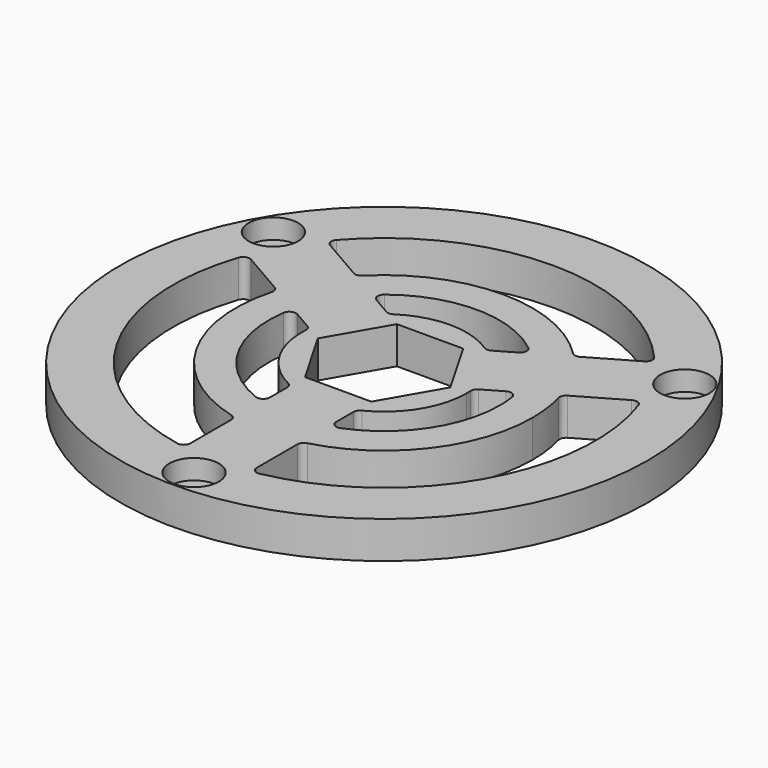
from build123d import *

# Parameters (mm, degrees)
F0_R     = 50.8
F1_DEPTH = 7.14375
F3_DEPTH = 7.14475
F4_R     = 1.27
F5_R     = 4.7625
F6_DEPTH = 3.81


with BuildPart() as f1:
    # F0 (on Top) → F1 (new body)
    with BuildSketch(Plane.XY):
        Circle(F0_R)
        Polygon((-12.7582862486, 0), (-6.3791431243, 11.049), (6.3791431243, 11.049), (12.7582862486, 0), (6.3791431243, -11.049), (-6.3791431243, -11.049), align=None, mode=Mode.SUBTRACT)
    extrude(amount=F1_DEPTH)

    # F2 (on face) → F3 (cut, through all)
    with BuildSketch(Plane.XY.offset(7.14375)):
        with BuildLine():
            Line((-6.3791431243, -40.1362197149), (-6.3791431243, -27.8538535575))
            ThreePointArc((-6.3791431243, -27.8538535575), (-24.7466759131, -14.2875), (-27.3117163362, 8.4024267787))
            Line((-27.3117163362, 8.4024267787), (-37.9485574471, 14.5436098574))
            ThreePointArc((-37.9485574471, 14.5436098574), (-35.1952724098, -20.32), (-6.3791431243, -40.1362197149))
        make_face()
        Polygon((-38.3481822298, 25.019), (-40.8411806922, 25.019), (-42.0876799234, 22.86), (-40.8411806922, 20.701), (-38.3481822298, 20.701), (-37.1016829987, 22.86), align=None)
        Polygon((1.2464992312, -43.561), (-1.2464992312, -43.561), (-2.4929984624, -45.72), (-1.2464992312, -47.879), (1.2464992312, -47.879), (2.4929984624, -45.72), align=None)
        Polygon((40.8411806922, 25.019), (38.3481822298, 25.019), (37.1016829987, 22.86), (38.3481822298, 20.701), (40.8411806922, 20.701), (42.0876799234, 22.86), align=None)
        with BuildLine():
            ThreePointArc((-20.9325732119, 19.4514267787), (0, 28.575), (20.9325732119, 19.4514267787))
            Line((20.9325732119, 19.4514267787), (31.5694143228, 25.5926098574))
            ThreePointArc((31.5694143228, 25.5926098574), (0, 40.64), (-31.5694143228, 25.5926098574))
            Line((-31.5694143228, 25.5926098574), (-20.9325732119, 19.4514267787))
        make_face()
        with BuildLine():
            Line((6.3791431243, -27.8538535575), (6.3791431243, -40.1362197149))
            ThreePointArc((6.3791431243, -40.1362197149), (35.1952724098, -20.32), (37.9485574471, 14.5436098574))
            Line((37.9485574471, 14.5436098574), (27.3117163362, 8.4024267787))
            ThreePointArc((27.3117163362, 8.4024267787), (28.2574142422, 4.2484309276), (28.575, 0))
            ThreePointArc((28.575, 0), (22.3474231152, -17.8079562306), (6.3791431243, -27.8538535575))
        make_face()
        with BuildLine():
            Line((6.3791431243, -14.5369239525), (6.3791431243, -21.2898369651))
            ThreePointArc((6.3791431243, -21.2898369651), (17.8287279543, -13.2697808773), (22.225, 0))
            ThreePointArc((22.225, 0), (22.0750217642, 2.5776033652), (21.6271112163, 5.1204184825))
            Line((21.6271112163, 5.1204184825), (15.7789169979, 1.7439619762))
            ThreePointArc((15.7789169979, 1.7439619762), (15.8509610488, 0.8733034006), (15.875, 0))
            ThreePointArc((15.875, 0), (13.2906832424, -8.6817834545), (6.3791431243, -14.5369239525))
        make_face()
        with BuildLine():
            Line((9.3997738736, 12.7929619762), (15.2479680921, 16.1694184825))
            ThreePointArc((15.2479680921, 16.1694184825), (0, 22.225), (-15.2479680921, 16.1694184825))
            Line((-15.2479680921, 16.1694184825), (-9.3997738736, 12.7929619762))
            ThreePointArc((-9.3997738736, 12.7929619762), (0, 15.875), (9.3997738736, 12.7929619762))
        make_face()
        with BuildLine():
            ThreePointArc((-21.6271112163, 5.1204184825), (-19.2474145991, -11.1125), (-6.3791431243, -21.2898369651))
            Line((-6.3791431243, -21.2898369651), (-6.3791431243, -14.5369239525))
            ThreePointArc((-6.3791431243, -14.5369239525), (-13.7481532851, -7.9375), (-15.7789169979, 1.7439619762))
            Line((-15.7789169979, 1.7439619762), (-21.6271112163, 5.1204184825))
        make_face()
    extrude(amount=-F3_DEPTH, mode=Mode.SUBTRACT)

    # F4
    f4_edges = [f1.edges().sort_by_distance(p)[0] for p in [
        (-37.948557, 14.54361, 3.571875),
        (-27.311716, 8.402427, 3.571875),
        (-6.379143, -40.13622, 3.571875),
        (-6.379143, -27.853854, 3.571875),
        (-21.627111, 5.120418, 3.571875),
        (-15.778917, 1.743962, 3.571875),
        (-6.379143, -21.289837, 3.571875),
        (-6.379143, -14.536924, 3.571875),
        (6.379143, -21.289837, 3.571875),
        (6.379143, -14.536924, 3.571875),
        (21.627111, 5.120418, 3.571875),
        (15.778917, 1.743962, 3.571875),
        (6.379143, -40.13622, 3.571875),
        (6.379143, -27.853854, 3.571875),
        (37.948557, 14.54361, 3.571875),
        (27.311716, 8.402427, 3.571875),
        (31.569414, 25.59261, 3.571875),
        (20.932573, 19.451427, 3.571875),
        (-31.569414, 25.59261, 3.571875),
        (-20.932573, 19.451427, 3.571875),
        (15.247968, 16.169418, 3.571875),
        (9.399774, 12.792962, 3.571875),
        (-15.247968, 16.169418, 3.571875),
        (-9.399774, 12.792962, 3.571875),
    ]]
    fillet(f4_edges, radius=F4_R)

    # F5 (on face) → F6 (cut)
    with BuildSketch(Plane.XY.offset(7.14375)):
        with Locations((-39.594681461, 22.86)):
            Circle(F5_R)
        Polygon((-42.0876799234, 22.86), (-40.8411806922, 25.019), (-38.3481822298, 25.019), (-37.1016829987, 22.86), (-38.3481822298, 20.701), (-40.8411806922, 20.701), align=None, mode=Mode.SUBTRACT)
        with Locations((39.594681461, 22.86)):
            Circle(F5_R)
        Polygon((38.3481822298, 25.019), (40.8411806922, 25.019), (42.0876799234, 22.86), (40.8411806922, 20.701), (38.3481822298, 20.701), (37.1016829987, 22.86), align=None, mode=Mode.SUBTRACT)
        with Locations((0, -45.72)):
            Circle(F5_R)
        Polygon((-2.4929984624, -45.72), (-1.2464992312, -43.561), (1.2464992312, -43.561), (2.4929984624, -45.72), (1.2464992312, -47.879), (-1.2464992312, -47.879), align=None, mode=Mode.SUBTRACT)
    extrude(amount=-F6_DEPTH, mode=Mode.SUBTRACT)


solid = f1.part
